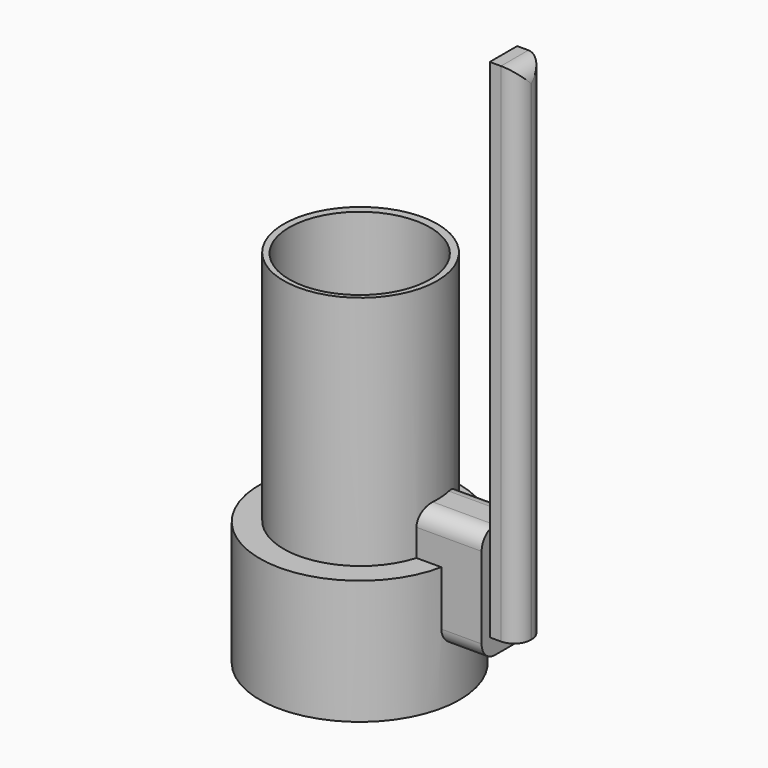
from build123d import *

# Parameters (mm, degrees)
F0_R      = 47.117
F1_DEPTH  = 220.98
F3_D      = 78.74
F4_R      = 61.2968374211
F5_DEPTH  = 76.2
F7_D      = 86.36
F8_W      = 33.8315991685
F8_H      = 70.290889591
F9_DEPTH  = 40.894
F10_R     = 10.16
F11_W     = 21.0215765983
F11_H     = 1.9707717001
F12_DEPTH = 17.018
F13_W     = 17.018
F13_H     = 21.0215765983
F14_DEPTH = 308.61
F15_R     = 10.16


with BuildPart() as f1:
    # F0 (on Top) → F1 (new body)
    with BuildSketch(Plane.XY):
        with Locations((-44.1687442362, -30.721032992)):
            Circle(F0_R)
    extrude(amount=F1_DEPTH)

    # F3 (through all)
    with Locations(Plane(origin=(0, 0, 0), x_dir=(1, 0, 0), z_dir=(0, 0, -1))):
        with Locations((-44.1687442362, 30.721032992)):
            Hole(F3_D / 2)

    # F4 (on Top) → F5 (join)
    with BuildSketch(Plane.XY):
        with Locations((-43.806668371, -31.8049825728)):
            Circle(F4_R)
    extrude(amount=F5_DEPTH)

    # F7 (through all)
    with Locations(Plane(origin=(0, 0, 0), x_dir=(1, 0, 0), z_dir=(0, 0, -1))):
        with Locations((-43.806668371, 31.8049825728)):
            Hole(F7_D / 2)

    # F8 (on Right) → F9 (join)
    with BuildSketch(Plane.YZ):
        with Locations((-27.3374826647, 67.7915308625)):
            Rectangle(F8_W, F8_H)
    extrude(amount=F9_DEPTH)

    # F10
    f10_edges = [f1.edges().sort_by_distance(p)[0] for p in [
        (20.447, -10.421683, 102.936976),
        (20.928586, -44.253282, 102.936976),
        (27.266726, -10.421683, 32.646086),
        (28.553423, -44.253282, 32.646086),
    ]]
    fillet(f10_edges, radius=F10_R)

    # F11 (on face) → F12 (join)
    with BuildSketch(Plane.YZ.offset(40.894)):
        with Locations((-27.5017125532, 44.7991844267)):
            Rectangle(F11_W, F11_H)
    extrude(amount=F12_DEPTH)

    # F13 (on face) → F14 (join)
    with BuildSketch(Plane.XY.offset(45.7845702767)):
        with Locations((49.403, -27.5017125532)):
            Rectangle(F13_W, F13_H)
    extrude(amount=F14_DEPTH)

    # F15
    f15_edges = [f1.edges().sort_by_distance(p)[0] for p in [
        (57.912, -38.012501, 199.104184),
        (57.912, -16.990924, 199.104184),
        (57.912, -27.501713, 354.39457),
    ]]
    fillet(f15_edges, radius=F15_R)


solid = f1.part
